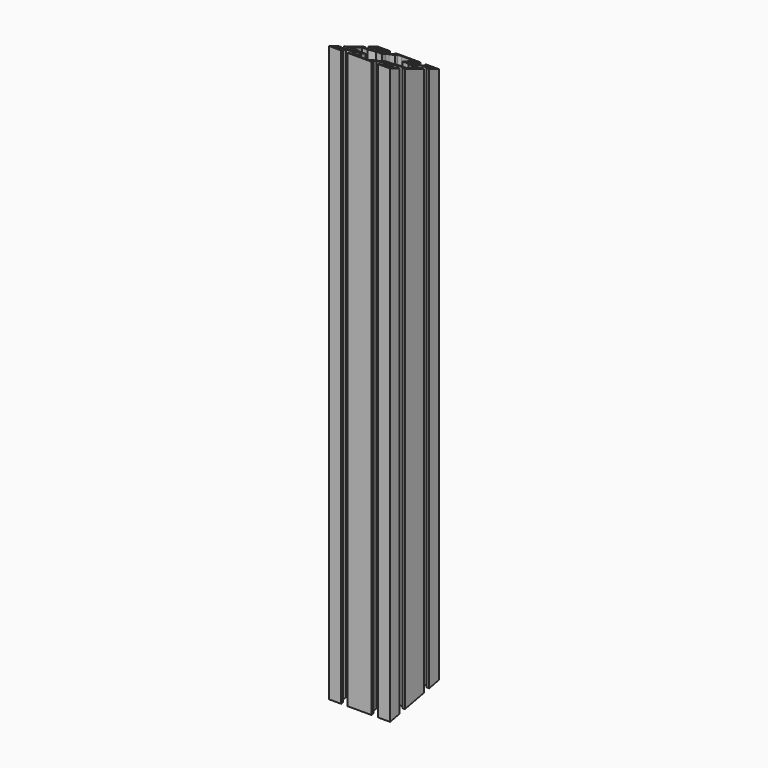
from build123d import *

# Parameters (mm, degrees)
F0_R          = 3
F0_R_2        = 2.5
F1_DEPTH      = 566.4
F2_R          = 2
F3_R          = 7
F6_DEPTH      = 30
F6_DEPTH_BACK = 30


# Not quite as in the source:
# - a feature names something its author has since deleted; it is built from what else it names


with BuildPart() as f1:
    # F0 (on Top) → F1 (new body)
    with BuildSketch(Plane.XY):
        with BuildLine():
            Line((18.15, -30), (30, -30))
            Line((30, -30), (30, -18.15))
            Line((30, -18.15), (27.5, -18.15))
            Line((27.5, -18.15), (27.5, -20.15))
            Line((27.5, -20.15), (21.5477069044, -20.15))
            ThreePointArc((21.5477069044, -20.15), (19.5, -15), (21.5477069044, -9.85))
            Line((21.5477069044, -9.85), (27.5, -9.85))
            Line((27.5, -9.85), (27.5, -11.85))
            Line((27.5, -11.85), (30, -11.85))
            Line((30, -11.85), (30, 11.85))
            Line((30, 11.85), (27.5, 11.85))
            Line((27.5, 11.85), (27.5, 9.85))
            Line((27.5, 9.85), (21.5477069044, 9.85))
            ThreePointArc((21.5477069044, 9.85), (19.5, 15), (21.5477069044, 20.15))
            Line((21.5477069044, 20.15), (27.5, 20.15))
            Line((27.5, 20.15), (27.5, 18.15))
            Line((27.5, 18.15), (30, 18.15))
            Line((30, 18.15), (30, 30))
            Line((30, 30), (18.15, 30))
            Line((18.15, 30), (18.15, 27.5))
            Line((18.15, 27.5), (20.15, 27.5))
            Line((20.15, 27.5), (20.15, 21.5477069044))
            ThreePointArc((20.15, 21.5477069044), (15, 19.5), (9.85, 21.5477069044))
            Line((9.85, 21.5477069044), (9.85, 27.5))
            Line((9.85, 27.5), (11.85, 27.5))
            Line((11.85, 27.5), (11.85, 30))
            Line((11.85, 30), (-11.85, 30))
            Line((-11.85, 30), (-11.85, 27.5))
            Line((-11.85, 27.5), (-9.85, 27.5))
            Line((-9.85, 27.5), (-9.85, 21.5477069044))
            ThreePointArc((-9.85, 21.5477069044), (-15, 19.5), (-20.15, 21.5477069044))
            Line((-20.15, 21.5477069044), (-20.15, 27.5))
            Line((-20.15, 27.5), (-18.15, 27.5))
            Line((-18.15, 27.5), (-18.15, 30))
            Line((-18.15, 30), (-30, 30))
            Line((-30, 30), (-30, 18.15))
            Line((-30, 18.15), (-27.5, 18.15))
            Line((-27.5, 18.15), (-27.5, 20.15))
            Line((-27.5, 20.15), (-21.5477069044, 20.15))
            ThreePointArc((-21.5477069044, 20.15), (-19.5, 15), (-21.5477069044, 9.85))
            Line((-21.5477069044, 9.85), (-27.5, 9.85))
            Line((-27.5, 9.85), (-27.5, 11.85))
            Line((-27.5, 11.85), (-30, 11.85))
            Line((-30, 11.85), (-30, -11.85))
            Line((-30, -11.85), (-27.5, -11.85))
            Line((-27.5, -11.85), (-27.5, -9.85))
            Line((-27.5, -9.85), (-21.5477069044, -9.85))
            ThreePointArc((-21.5477069044, -9.85), (-19.5, -15), (-21.5477069044, -20.15))
            Line((-21.5477069044, -20.15), (-27.5, -20.15))
            Line((-27.5, -20.15), (-27.5, -18.15))
            Line((-27.5, -18.15), (-30, -18.15))
            Line((-30, -18.15), (-30, -30))
            Line((-30, -30), (-18.15, -30))
            Line((-18.15, -30), (-18.15, -27.5))
            Line((-18.15, -27.5), (-20.15, -27.5))
            Line((-20.15, -27.5), (-20.15, -21.5477069044))
            ThreePointArc((-20.15, -21.5477069044), (-15, -19.5), (-9.85, -21.5477069044))
            Line((-9.85, -21.5477069044), (-9.85, -27.5))
            Line((-9.85, -27.5), (-11.85, -27.5))
            Line((-11.85, -27.5), (-11.85, -30))
            Line((-11.85, -30), (11.85, -30))
            Line((11.85, -30), (11.85, -27.5))
            Line((11.85, -27.5), (9.85, -27.5))
            Line((9.85, -27.5), (9.85, -21.5477069044))
            ThreePointArc((9.85, -21.5477069044), (15, -19.5), (20.15, -21.5477069044))
            Line((20.15, -21.5477069044), (20.15, -27.5))
            Line((20.15, -27.5), (18.15, -27.5))
            Line((18.15, -27.5), (18.15, -30))
        make_face()
        with Locations((-25, -25)):
            Circle(F0_R, mode=Mode.SUBTRACT)
        with Locations((-15, -15)):
            Circle(F0_R_2, mode=Mode.SUBTRACT)
        with Locations((25, -25)):
            Circle(F0_R, mode=Mode.SUBTRACT)
        with Locations((15, -15)):
            Circle(F0_R_2, mode=Mode.SUBTRACT)
        with Locations((-25, 25)):
            Circle(F0_R, mode=Mode.SUBTRACT)
        with Locations((-15, 15)):
            Circle(F0_R_2, mode=Mode.SUBTRACT)
        Polygon((-7, 22), (-7, 27.5), (0, 27.5), (7, 27.5), (7, 22), (10, 16), (10, 10), (16, 10), (22, 7), (27.5, 7), (27.5, 0), (27.5, -7), (22, -7), (16, -10), (10, -10), (10, -16), (7, -22), (7, -27.5), (0, -27.5), (-7, -27.5), (-7, -22), (-10, -16), (-10, -10), (-16, -10), (-22, -7), (-27.5, -7), (-27.5, 0), (-27.5, 7), (-22, 7), (-16, 10), (-10, 10), (-10, 16), align=None, mode=Mode.SUBTRACT)
        with Locations((15, 15)):
            Circle(F0_R_2, mode=Mode.SUBTRACT)
        with Locations((25, 25)):
            Circle(F0_R, mode=Mode.SUBTRACT)
    extrude(amount=F1_DEPTH)

    # F2
    f2_edges = [f1.edges().sort_by_distance(p)[0] for p in [
        (-7, 27.5, 283.2),
        (7, 27.5, 283.2),
    ]]
    fillet(f2_edges, radius=F2_R)

    # F3
    f3_edges = [f1.edges().sort_by_distance(p)[0] for p in [
        (-10, 16, 283.2),
        (10, 16, 283.2),
    ]]
    fillet(f3_edges, radius=F3_R)

    # F5 (on Right) → F6 (cut, two sides)
    with BuildSketch(Plane.YZ) as f6_sk:
        Polygon((-5.9431682558, -120.9418602831), (191.6672123159, -81.6347116648), (167.6103805717, 39.3071486183), (-30, 0), align=None)
        Polygon((112.1150393779, 507.5340232725), (142.1183047075, 579.9683133465), (0.0032653295, 638.834290074), (-30, 566.4), align=None)
    extrude(amount=F6_DEPTH, mode=Mode.SUBTRACT)
    extrude(f6_sk.sketch, amount=-F6_DEPTH_BACK, mode=Mode.SUBTRACT)


solid = f1.part
